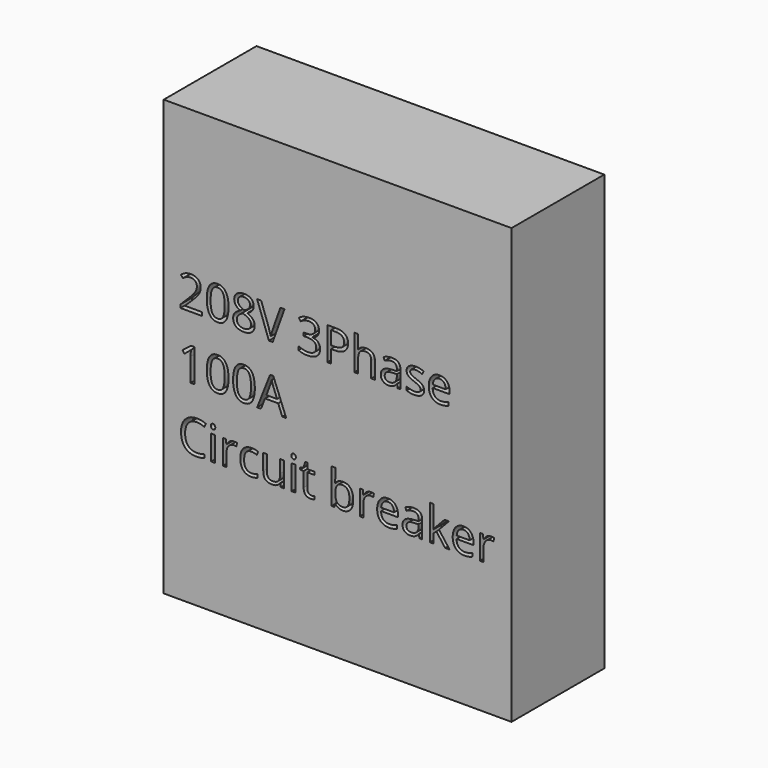
from build123d import *

# Parameters (mm, degrees)
F0_W         = 609.6
F0_H         = 762
F1_DEPTH     = 203.2
F2_TEXT_SIZE = 80.6240137067
F3_DEPTH     = 25.4


# Not quite as in the source:
# - Text() gives the source's letters only with a copy of the font that has no kerning and outlines rounded to 1/6400 em; it was checked with that copy


with BuildPart() as f1:
    # F0 (on Front) → F1 (new body)
    with BuildSketch(Plane.XZ):
        Rectangle(F0_W, F0_H)
    extrude(amount=F1_DEPTH)

    # F2 (on face) → F3 (cut)
    with BuildSketch(Plane.XZ.offset(203.2)):
        with Locations((-279.4, 68.9507101312)):
            Text('208V 3Phase', F2_TEXT_SIZE, font='Open Sans', text_align=(TextAlign.LEFT, TextAlign.BOTTOM))
        with Locations((-279.4, -40.6979485099)):
            Text('100A', F2_TEXT_SIZE, font='Open Sans', text_align=(TextAlign.LEFT, TextAlign.BOTTOM))
        with Locations((-279.4, -150.3466071509)):
            Text('Circuit breaker', F2_TEXT_SIZE, font='Open Sans', text_align=(TextAlign.LEFT, TextAlign.BOTTOM))
    extrude(amount=-F3_DEPTH, mode=Mode.SUBTRACT)


solid = f1.part
